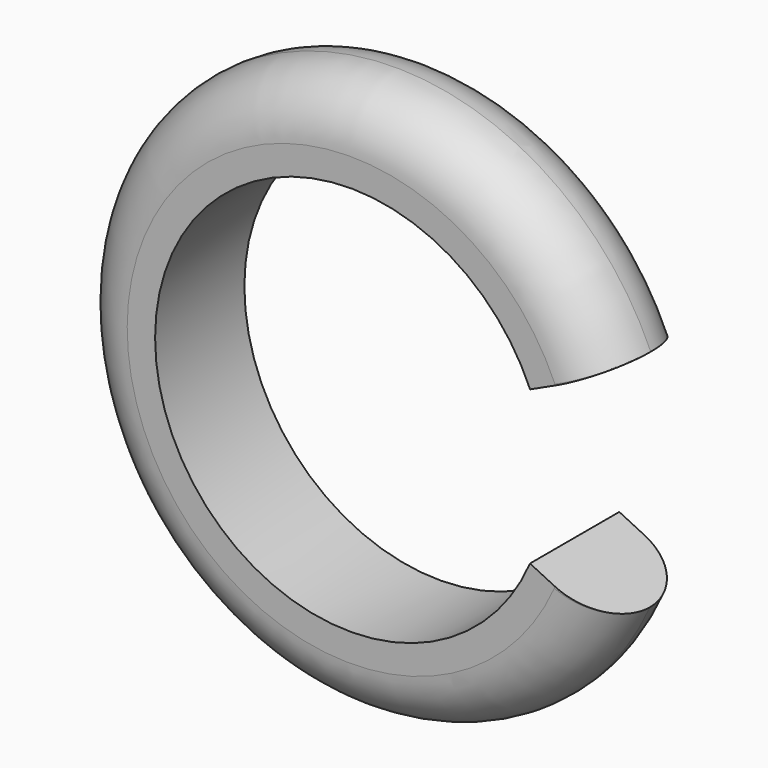
from build123d import *

# Parameters (mm, degrees)
F1_DEPTH = 1
F2_R     = 0.49999
F3_DEPTH = 25


# Not quite as in the source:
# - a fillet or chamfer is up to 0.001 mm smaller than in the source, because OpenCascade refuses the exact size


with BuildPart() as f1:
    # F0 (on Front) → F1 (new body)
    with BuildSketch(Plane.XZ):
        with BuildLine():
            Line((1.6101524701, 0.6854991051), (2.2910968404, 1.0004375382))
            ThreePointArc((2.2910968404, 1.0004375382), (-2.4999847011, 0.0087461138), (2.2840408488, -1.016443506))
            Line((2.2840408488, -1.016443506), (1.6091022659, -0.6879606804))
            ThreePointArc((1.6091022659, -0.6879606804), (-1.7499994884, 0.001338122), (1.6101524701, 0.6854991051))
        make_face()
        with BuildLine():
            ThreePointArc((2.2840408488, -1.016443506), (2.4454142923, -0.5195661065), (2.5, 0))
            ThreePointArc((2.5, 0), (2.4472170011, 0.5110077783), (2.2910968404, 1.0004375382))
            Line((2.2910968404, 1.0004375382), (1.6101524701, 0.6854991051))
            ThreePointArc((1.6101524701, 0.6854991051), (1.714681723, 0.3498093605), (1.75, 0))
            ThreePointArc((1.75, 0), (1.7144137431, -0.3511203744), (1.6091022659, -0.6879606804))
            Line((1.6091022659, -0.6879606804), (2.2840408488, -1.016443506))
        make_face()
    extrude(amount=F1_DEPTH)

    # F2 (radius 0.5 in the source; OpenCascade refuses exactly that, so slightly less here)
    f2_edges = [f1.edges().sort_by_distance(p)[0] for p in [
        (-2.284041, -1, 1.016444),
        (-2.284041, 0, 1.016444),
    ]]
    fillet(f2_edges, radius=F2_R)

    # F0 (on Front) → F3 (cut)
    with BuildSketch(Plane.XZ):
        with BuildLine():
            ThreePointArc((2.2840408488, -1.016443506), (2.4454142923, -0.5195661065), (2.5, 0))
            ThreePointArc((2.5, 0), (2.4472170011, 0.5110077783), (2.2910968404, 1.0004375382))
            Line((2.2910968404, 1.0004375382), (1.6101524701, 0.6854991051))
            ThreePointArc((1.6101524701, 0.6854991051), (1.714681723, 0.3498093605), (1.75, 0))
            ThreePointArc((1.75, 0), (1.7144137431, -0.3511203744), (1.6091022659, -0.6879606804))
            Line((1.6091022659, -0.6879606804), (2.2840408488, -1.016443506))
        make_face()
    extrude(amount=F3_DEPTH, mode=Mode.SUBTRACT)


solid = f1.part
